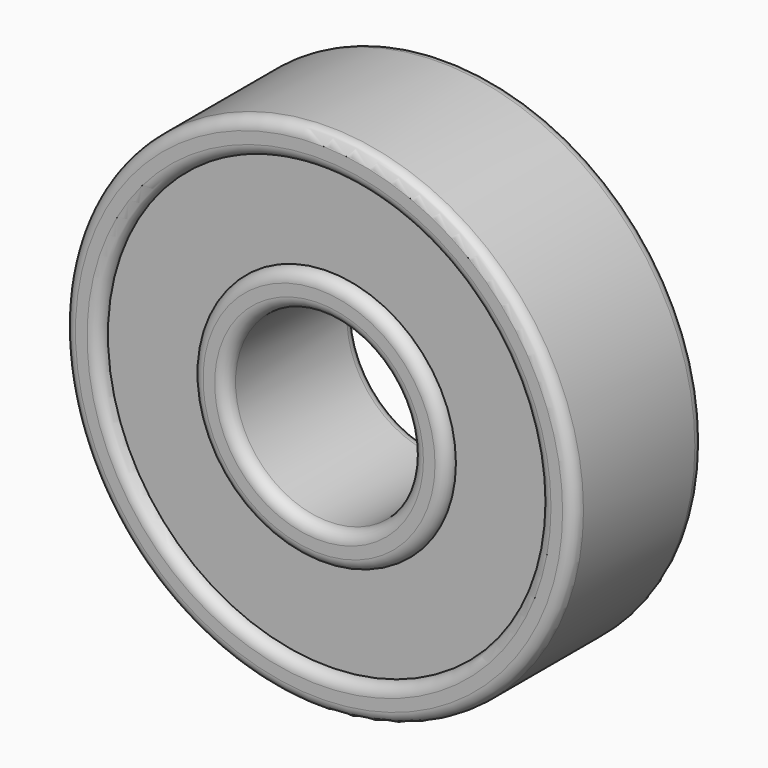
from build123d import *

# Parameters (mm, degrees)
F0_R     = 11
F0_R_2   = 9.5
F1_DEPTH = 3.5
F0_R_3   = 5.5
F0_R_4   = 4
F2_DEPTH = 3
F3_R     = 0.49999


# Not quite as in the source:
# - a fillet or chamfer is up to 0.001 mm smaller than in the source, because OpenCascade refuses the exact size


with BuildPart() as f1:
    # F0 (on Front) → F1 (new body, symmetric)
    with BuildSketch(Plane.XZ):
        Circle(F0_R)
        Circle(F0_R_2, mode=Mode.SUBTRACT)
    extrude(amount=F1_DEPTH, both=True)



with BuildPart() as f1b:
    # F0 (on Front) → F1, piece 2 (new body, symmetric)
    with BuildSketch(Plane.XZ):
        Circle(F0_R_3)
        Circle(F0_R_4, mode=Mode.SUBTRACT)
    extrude(amount=F1_DEPTH, both=True)


with BuildPart() as f1_1:
    add(f1.part)

    add(f1b.part)  # F2 merges F1b
    # F0 (on Front) → F2 (join, symmetric)
    with BuildSketch(Plane.XZ):
        Circle(F0_R_2)
        Circle(F0_R_3, mode=Mode.SUBTRACT)
    extrude(amount=F2_DEPTH, both=True)

    # F3 (radius 0.5 in the source; OpenCascade refuses exactly that, so slightly less here)
    f3_edges = [f1_1.edges().sort_by_distance(p)[0] for p in [
        (-11, -3.5, 0),
        (-9.5, -3.5, 0),
        (-5.5, -3.5, 0),
        (-4, -3.5, 0),
        (-11, 3.5, 0),
        (-9.5, 3.5, 0),
        (-5.5, 3.5, 0),
        (-4, 3.5, 0),
    ]]
    fillet(f3_edges, radius=F3_R)


solid = f1_1.part
